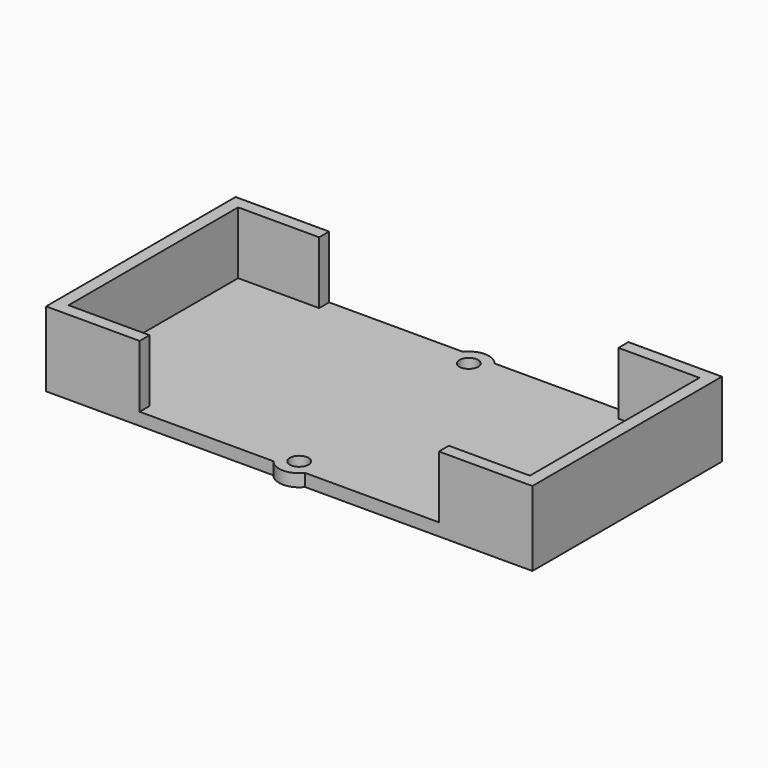
from build123d import *

# Parameters (mm, degrees)
F1_DEPTH = 2
F3_DEPTH = 10
F5_D     = 3


with BuildPart() as f1:
    # F0 (on Top) → F1 (new body)
    with BuildSketch(Plane.XY):
        with BuildLine():
            Line((0, 38), (0, 0))
            Line((0, 0), (36.4592920615, 0))
            ThreePointArc((36.4592920615, 0), (36.0912119201, 3.4121433125), (39, 5.2334496794))
            Line((39, 5.2334496794), (39, 32.7665503206))
            ThreePointArc((39, 32.7665503206), (36.0912119201, 34.5878566875), (36.4592920615, 38))
            Line((36.4592920615, 38), (0, 38))
        make_face()
        with BuildLine():
            ThreePointArc((39, 5.2334496794), (36.0912119201, 3.4121433125), (36.4592920615, 0))
            Line((36.4592920615, 0), (39, 0))
            Line((39, 0), (39, 5.2334496794))
        make_face()
        with BuildLine():
            Line((39, 0), (36.4592920615, 0))
            ThreePointArc((36.4592920615, 0), (39, -1.2334496794), (41.5407079385, 0))
            Line((41.5407079385, 0), (39, 0))
        make_face()
        with BuildLine():
            Line((39, 5.2334496794), (39, 0))
            Line((39, 0), (41.5407079385, 0))
            ThreePointArc((41.5407079385, 0), (42.0553598886, 0.941712336), (42.2334496794, 2))
            ThreePointArc((42.2334496794, 2), (41.2863941949, 4.2863941949), (39, 5.2334496794))
        make_face()
        with BuildLine():
            Line((39, 32.7665503206), (39, 5.2334496794))
            ThreePointArc((39, 5.2334496794), (41.2863941949, 4.2863941949), (42.2334496794, 2))
            ThreePointArc((42.2334496794, 2), (42.0553598886, 0.941712336), (41.5407079385, 0))
            Line((41.5407079385, 0), (78, 0))
            Line((78, 0), (78, 38))
            Line((78, 38), (41.5407079385, 38))
            ThreePointArc((41.5407079385, 38), (42.0553598886, 37.058287664), (42.2334496794, 36))
            ThreePointArc((42.2334496794, 36), (41.2863941949, 33.7136058051), (39, 32.7665503206))
        make_face()
        with BuildLine():
            ThreePointArc((41.5407079385, 38), (39, 39.2334496794), (36.4592920615, 38))
            Line((36.4592920615, 38), (39, 38))
            Line((39, 38), (41.5407079385, 38))
        make_face()
        with BuildLine():
            Line((39, 38), (36.4592920615, 38))
            ThreePointArc((36.4592920615, 38), (36.0912119201, 34.5878566875), (39, 32.7665503206))
            Line((39, 32.7665503206), (39, 38))
        make_face()
        with BuildLine():
            Line((39, 38), (39, 32.7665503206))
            ThreePointArc((39, 32.7665503206), (41.2863941949, 33.7136058051), (42.2334496794, 36))
            ThreePointArc((42.2334496794, 36), (42.0553598886, 37.058287664), (41.5407079385, 38))
            Line((41.5407079385, 38), (39, 38))
        make_face()
    extrude(amount=F1_DEPTH)

    # F2 (on face) → F3 (join)
    with BuildSketch(Plane.XY.offset(2)):
        Polygon((2, 36), (15, 36), (15, 38), (0, 38), (0, 0), (15, 0), (15, 2), (2, 2), align=None)
        Polygon((78, 38), (63, 38), (63, 36), (76, 36), (76, 2), (63, 2), (63, 0), (78, 0), align=None)
    extrude(amount=F3_DEPTH)

    # F5 (through all)
    with Locations(Plane(origin=(0, 0, 0), x_dir=(1, 0, 0), z_dir=(0, 0, -1))):
        with Locations((39, -2), (39, -36)):
            Hole(F5_D / 2)


solid = f1.part
